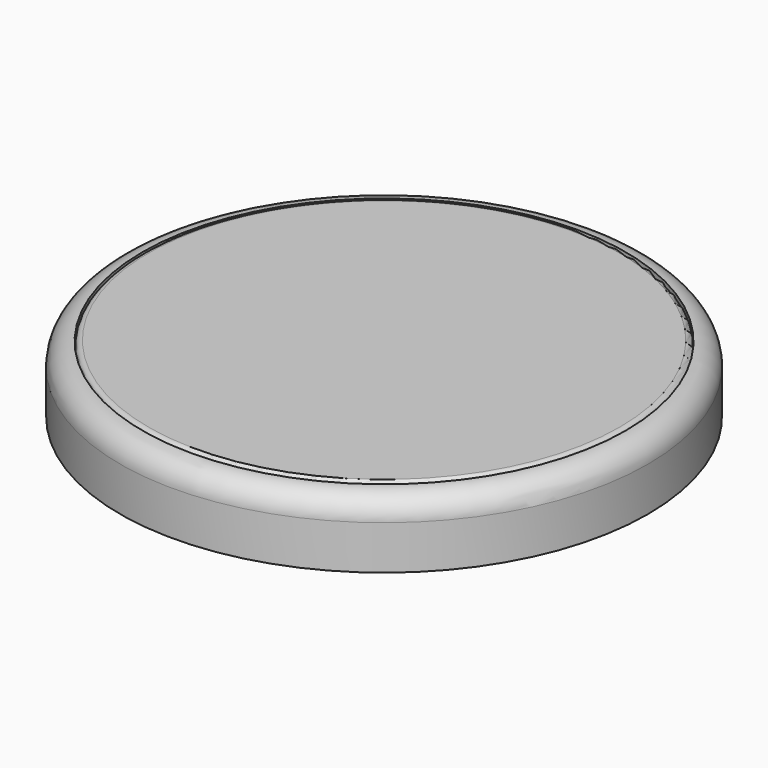
from build123d import *

# Parameters (mm, degrees)
F0_R         = 4.74
F1_DEPTH     = 1.19
F2_R         = 0.4
F3_T         = -0.1
F4_R         = 4.3315
F5_DEPTH     = 1.11
F6_R         = 0.1
F7_TEXT_SIZE = 4.1681468324
F8_DEPTH     = 0.1


# Not quite as in the source:
# - a shell that OpenCascade refuses in one call is made with other operations: the cavity is built on its own and cut out
# - Text() gives the source's letters only with a copy of the font that has no kerning and outlines rounded to 1/6400 em; it was checked with that copy


with BuildPart() as f1:
    # F0 (on Top) → F1 (new body)
    with BuildSketch(Plane.XY):
        Circle(F0_R)
    extrude(amount=F1_DEPTH)

    # F2
    f2_edges = [f1.edges().sort_by_distance(p)[0] for p in [
        (-4.74, 0, 1.19),
    ]]
    fillet(f2_edges, radius=F2_R)

    # F3: a shell. OpenCascade refuses it in one call, so the cavity is built on its own and cut out:
    # the body offset inwards by the wall thickness, plus a prism from it out through each open face.
    f3_core = offset(f1.part, amount=F3_T, mode=Mode.PRIVATE)
    f3_exits = [f3_core.faces().sort_by_distance(p)[0] for p in [
        (0, 0, 1.09),
    ]]
    add(f3_core, mode=Mode.SUBTRACT)
    extrude(f3_exits, amount=-F3_T, mode=Mode.SUBTRACT)

    # F4 (on face) → F5 (join)
    with BuildSketch(Plane.XY.offset(0.1)):
        Circle(F4_R)
    extrude(amount=F5_DEPTH)

    # F6
    f6_edges = [f1.edges().sort_by_distance(p)[0] for p in [
        (-4.3315, 0, 1.21),
    ]]
    fillet(f6_edges, radius=F6_R)

    # F7 (on face) → F8 (cut)
    with BuildSketch(Plane(origin=(0, 0, 0), x_dir=(1, 0, 0), z_dir=(0, 0, -1))):
        with Locations((-1.1, 1.0997209374)):
            Text('+', F7_TEXT_SIZE, font='Open Sans', font_style=FontStyle.BOLD, text_align=(TextAlign.LEFT, TextAlign.BOTTOM))
    extrude(amount=-F8_DEPTH, mode=Mode.SUBTRACT)


solid = f1.part
